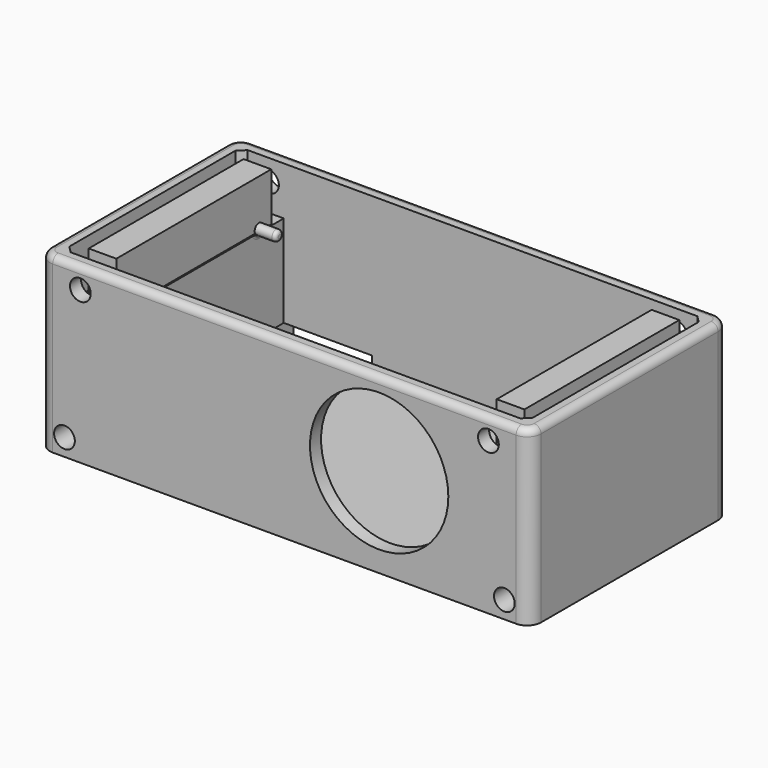
from build123d import *

# Parameters (mm, degrees)
F0_W         = 71
F0_H         = 36
F1_DEPTH     = 2
F2_W         = 71
F2_H         = 36
F2_W_2       = 67
F2_H_2       = 32
F3_DEPTH     = 23
F4_SIZE      = 1
F5_R         = 2
F6_R         = 1
F7_W         = 6.2
F7_H         = 32
F7_H_2       = 34
F8_DEPTH     = 16
F9_R         = 1.5
F10_DEPTH    = 36.001
F12_DEPTH    = 7
F13_R        = 1.5
F14_DEPTH    = 36.001
F17_R        = 10
F18_DEPTH    = 34
F19_R        = 1.25
F20_DEPTH    = 4
F21_R        = 1
F23_R        = 0.75
F24_DEPTH    = 3
F25_T4_ANGLE = 287.4532878227
F25_T9_ANGLE = 287.4532878227
F26_W        = 13
F26_H        = 2.7
F27_DEPTH    = 25


# Not quite as in the source:
# - a fillet or chamfer that OpenCascade refuses, or shapes differently, is made with other operations: its cross-section is extruded or revolved along the edge and cut away or added


with BuildPart() as f1:
    # F0 (on Top) → F1 (new body)
    with BuildSketch(Plane.XY):
        with Locations((35.5, -18)):
            Rectangle(F0_W, F0_H)
    extrude(amount=F1_DEPTH)

    # F2 (on face) → F3 (join)
    with BuildSketch(Plane.XY.offset(2)):
        with Locations((35.5, -18)):
            Rectangle(F2_W, F2_H)
        with Locations((35.5, -18)):
            Rectangle(F2_W_2, F2_H_2, mode=Mode.SUBTRACT)
    extrude(amount=F3_DEPTH)

    # F4
    f4_edges = [f1.edges().sort_by_distance(p)[0] for p in [
        (2, -2, 13.5),
        (2, -34, 13.5),
        (69, -2, 13.5),
        (69, -34, 13.5),
    ]]
    chamfer(f4_edges, length=F4_SIZE)

    # F5
    f5_edges = [f1.edges().sort_by_distance(p)[0] for p in [
        (0, -36, 12.5),
        (71, -36, 12.5),
        (71, 0, 12.5),
        (0, 0, 12.5),
    ]]
    fillet(f5_edges, radius=F5_R)

    # F6
    f6_edges = [f1.edges().sort_by_distance(p)[0] for p in [
        (0, -18, 25),
        (35.5, -36, 25),
        (71, -18, 25),
        (35.5, 0, 25),
    ]]
    fillet(f6_edges, radius=F6_R)

    # F7 (on face) → F8 (join)
    with BuildSketch(Plane.XY.offset(2)):
        with Locations((5.1, -18)):
            Rectangle(F7_W, F7_H)
        with Locations((65.9, -19)):
            Rectangle(F7_W, F7_H_2)
    extrude(amount=F8_DEPTH)

    # F9 (on face) → F10 (cut, through all)
    with BuildSketch(Plane.XZ.offset(36)):
        with Locations((3.7, 2.5)):
            Circle(F9_R)
        with Locations((67.3, 2.5)):
            Circle(F9_R)
    extrude(amount=-F10_DEPTH, mode=Mode.SUBTRACT)

    # F11 (on face) → F12 (join)
    with BuildSketch(Plane.XY.offset(18)):
        Polygon((8, -21.2), (8, -4), (4, -4), (4, -21.2), (4, -32), (8, -32), align=None)
        Polygon((67, -4), (63, -4), (63, -22), (63, -32), (67, -32), (67, -22), align=None)
    extrude(amount=F12_DEPTH)

    # F13 (on face) → F14 (cut, through all)
    with BuildSketch(Plane.XZ.offset(36)):
        with Locations((6, 22)):
            Circle(F13_R)
        with Locations((65, 22)):
            Circle(F13_R)
    extrude(amount=-F14_DEPTH, mode=Mode.SUBTRACT)

    # F17 (on face) → F18 (cut, through all)
    with BuildSketch(Plane.XZ.offset(36)):
        with Locations((49.2, 13)):
            Circle(F17_R)
    extrude(amount=-F18_DEPTH, mode=Mode.SUBTRACT)

    # F19 (on face) → F20 (join)
    with BuildSketch(Plane(origin=(0, -34, 0), x_dir=(-1, 0, 0), z_dir=(0, 1, 0))):
        with Locations((-58.7, 20.5)):
            Circle(F19_R)
        with Locations((-31.7, 20.5)):
            Circle(F19_R)
        with Locations((-31.7, 5.5)):
            Circle(F19_R)
        with Locations((-58.7, 5.5)):
            Circle(F19_R)
    extrude(amount=F20_DEPTH)

    # F21
    f21_edges = [f1.edges().sort_by_distance(p)[0] for p in [
        (57.45, -32, 20.5),
        (59.95, -34, 20.5),
        (59.95, -30, 20.5),
        (57.45, -32, 5.5),
        (59.95, -34, 5.5),
        (59.95, -30, 5.5),
        (30.45, -32, 20.5),
        (32.95, -34, 20.5),
        (32.95, -30, 20.5),
        (30.45, -32, 5.5),
        (32.95, -34, 5.5),
        (32.95, -30, 5.5),
    ]]
    fillet(f21_edges, radius=F21_R)

    # F23 (on face) → F24 (join)
    with BuildSketch(Plane.YZ.offset(8.2)):
        with Locations((-29.5, 18.5)):
            Circle(F23_R)
        with Locations((-6.5, 18.5)):
            Circle(F23_R)
    extrude(amount=F24_DEPTH)

    # F25: fillet of radius 0.5 on 6 edges, made by hand


with BuildPart() as f25_tool2:
    # F25_s3 → F25_t4 (revolve)
    with BuildSketch(Plane(origin=(0, -10.3497936524, -7.5952718618), x_dir=(1, 0, 0), z_dir=(0, 0.8062034954, 0.5916383388))):
        with BuildLine():
            ThreePointArc((8.7, -33.1180956607), (8.3464466094, -33.2645422701), (8.2, -33.6180956607))
            Line((8.2, -33.6180956607), (8.2, -33.1180956607))
            Line((8.2, -33.1180956607), (8.7, -33.1180956607))
        make_face()
    revolve(axis=Axis((8.2, -29.5, 18.5), (1, 0, 0)), revolution_arc=F25_T4_ANGLE)

    split(bisect_by=Plane.XY.offset(18), keep=Keep.BOTTOM)


with BuildPart() as f1_1:
    add(f1.part)

    # F25_t1: union F25_tool2
    add(f25_tool2.part)


with BuildPart() as f25_tool7:
    # F25_s8 → F25_t9 (revolve)
    with BuildSketch(Plane(origin=(0, 4.5993800964, 3.3752887643), x_dir=(1, 0, 0), z_dir=(0, 0.8062034954, 0.5916383388))):
        with BuildLine():
            ThreePointArc((8.7, -19.5104138677), (8.3464466094, -19.6568604771), (8.2, -20.0104138677))
            Line((8.2, -20.0104138677), (8.2, -19.5104138677))
            Line((8.2, -19.5104138677), (8.7, -19.5104138677))
        make_face()
    revolve(axis=Axis((8.2, -6.5, 18.5), (1, 0, 0)), revolution_arc=F25_T9_ANGLE)

    split(bisect_by=Plane.XY.offset(18), keep=Keep.BOTTOM)


with BuildPart() as f1_2:
    add(f1_1.part)

    # F25_t6: union F25_tool7
    add(f25_tool7.part)

    # F25_s11 → F25_t12 (revolve, cut)
    with BuildSketch(Plane.XY.offset(18.5)):
        with BuildLine():
            ThreePointArc((10.7, -28.75), (11.0535533906, -28.8964466094), (11.2, -29.25))
            Line((11.2, -29.25), (11.2, -28.75))
            Line((11.2, -28.75), (10.7, -28.75))
        make_face()
    revolve(axis=Axis((11.2, -29.5, 18.5), (1, 0, 0)), mode=Mode.SUBTRACT)

    # F25_s13 → F25_t14 (revolve, cut)
    with BuildSketch(Plane.XY.offset(18.5)):
        with BuildLine():
            ThreePointArc((10.7, -5.75), (11.0535533906, -5.8964466094), (11.2, -6.25))
            Line((11.2, -6.25), (11.2, -5.75))
            Line((11.2, -5.75), (10.7, -5.75))
        make_face()
    revolve(axis=Axis((11.2, -6.5, 18.5), (1, 0, 0)), mode=Mode.SUBTRACT)

    # F26 (on face) → F27 (cut)
    with BuildSketch(Plane(origin=(0, 0, 0), x_dir=(-1, 0, 0), z_dir=(0, 1, 0))):
        with Locations((-14.5, 3.35)):
            Rectangle(F26_W, F26_H)
    extrude(amount=-F27_DEPTH, mode=Mode.SUBTRACT)


solid = f1_2.part
